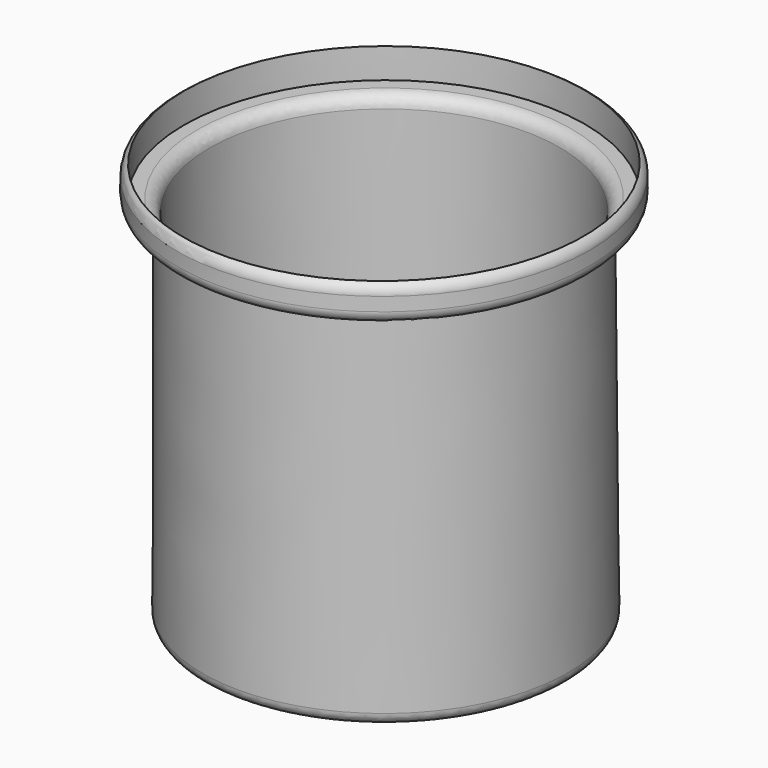
from build123d import *

# Parameters (mm, degrees)
F2_T = -2.54
F4_R = 5.08
F5_R = 5.08


# Not quite as in the source:
# - a fillet or chamfer that OpenCascade refuses, or shapes differently, is made with other operations: its cross-section is extruded or revolved along the edge and cut away or added
# - a feature of the source that left no trace in its solid (it failed there, or was rolled back) is left out


with BuildPart() as f1:
    # F0 (on Front) → F1 (revolve)
    with BuildSketch(Plane.XZ):
        Polygon((0.8919350803, -92.1029001474), (0.8186959634, -77.028170228), (-43.8721254468, -77.028170228), (-43.8721254468, -92.1029001474), align=None)
        Polygon((0.0736342535, 76.3270929456), (-75.8807361126, 76.3270929456), (-75.8807361126, -77.028170228), (-43.8721254468, -77.028170228), (0.8186959634, -77.028170228), align=None)
        Polygon((-86.4892601967, 76.3270929456), (-75.8807361126, 76.3270929456), (0.0736342535, 76.3270929456), (0, 91.4831534028), (-86.4892601967, 91.4831534028), align=None)
    revolve(axis=Axis((0.4459675401, 0, -0.3098733723), (0.0048583459, 0, -0.9999881982)))

    # F2
    f2_openings = [f1.faces().sort_by_distance(p)[0] for p in [
        (43.242589, 0, 91.903343),
    ]]
    offset(amount=F2_T, openings=f2_openings, kind=Kind.INTERSECTION)

    # F3: fillet of radius 5.08 on 2 edges, made by hand

    # F3_s1 → F3_t2 (revolve, cut)
    with BuildSketch(Plane.XZ):
        with BuildLine():
            ThreePointArc((-86.4892601967, 87.0837443516), (-85.8086692479, 89.6237443516), (-83.9492601967, 91.4831534028))
            Line((-83.9492601967, 91.4831534028), (-86.4892601967, 91.4831534028))
            Line((-86.4892601967, 91.4831534028), (-86.4892601967, 87.0837443516))
        make_face()
    revolve(axis=Axis((-0.0020414514, 0, 91.9033431879), (0.0048583459, 0, -0.9999881982)), mode=Mode.SUBTRACT)

    # F3_s3 → F3_t4 (revolve, cut)
    with BuildSketch(Plane.XZ):
        with BuildLine():
            ThreePointArc((-86.4892601967, 81.4070929456), (-85.0013626451, 77.8149904971), (-81.4092601967, 76.3270929456))
            Line((-81.4092601967, 76.3270929456), (-86.4892601967, 76.3270929456))
            Line((-86.4892601967, 76.3270929456), (-86.4892601967, 81.4070929456))
        make_face()
    revolve(axis=Axis((0.071591064, 0, 76.7476404672), (0.0048583459, 0, -0.9999881982)), mode=Mode.SUBTRACT)

    # F4
    f4_edges = [f1.edges().sort_by_distance(p)[0] for p in [
        (77.514507, 0, -76.282914),
        (45.653882, 0, -91.667947),
    ]]
    fillet(f4_edges, radius=F4_R)

    # F5
    f5_edges = [f1.edges().sort_by_distance(p)[0] for p in [
        (73.459859, 0, 79.580309),
        (74.949947, 0, -73.767714),
        (42.942847, 0, -74.078728),
        (43.089322, 0, -89.152747),
    ]]
    fillet(f5_edges, radius=F5_R)


solid = f1.part
